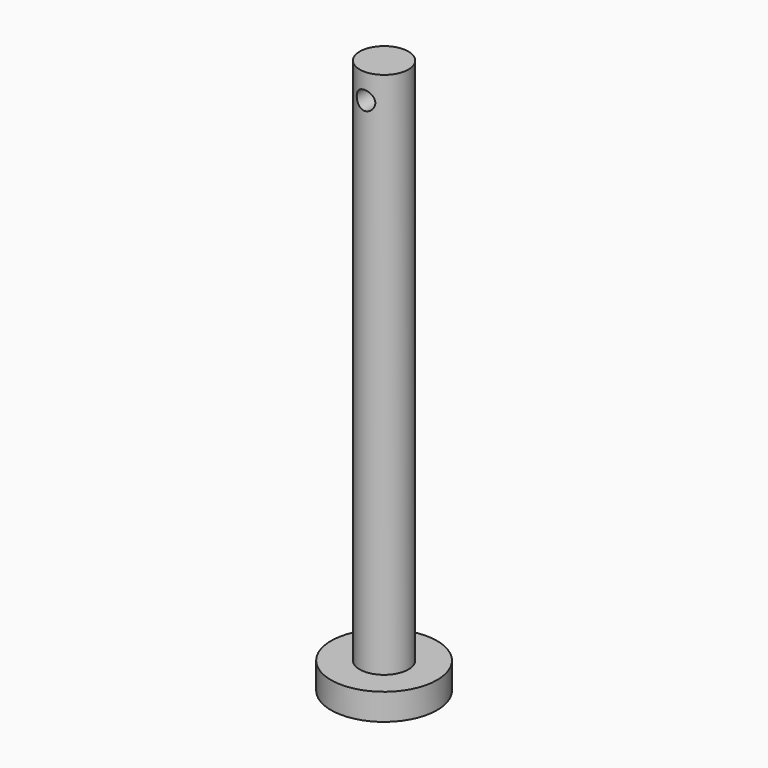
from build123d import *

# Parameters (mm, degrees)
F0_R     = 2.335
F1_DEPTH = 50.5726954
F2_R     = 5.08
F2_R_2   = 2.335
F3_DEPTH = 2.54
F4_R     = 0.889
F5_DEPTH = 12.7


with BuildPart() as f1:
    # F0 (on Top) → F1 (new body)
    with BuildSketch(Plane.XY):
        Circle(F0_R)
    extrude(amount=F1_DEPTH)

    # F2 (on face) → F3 (join)
    with BuildSketch(Plane(origin=(0, 0, 0), x_dir=(1, 0, 0), z_dir=(0, 0, -1))):
        Circle(F2_R)
        Circle(F2_R_2, mode=Mode.SUBTRACT)
        Circle(F2_R_2)
    extrude(amount=F3_DEPTH)

    # F4 (on Front) → F5 (cut, symmetric)
    with BuildSketch(Plane.XZ):
        with Locations((0, 48.1596954)):
            Circle(F4_R)
    extrude(amount=F5_DEPTH, both=True, mode=Mode.SUBTRACT)


solid = f1.part
